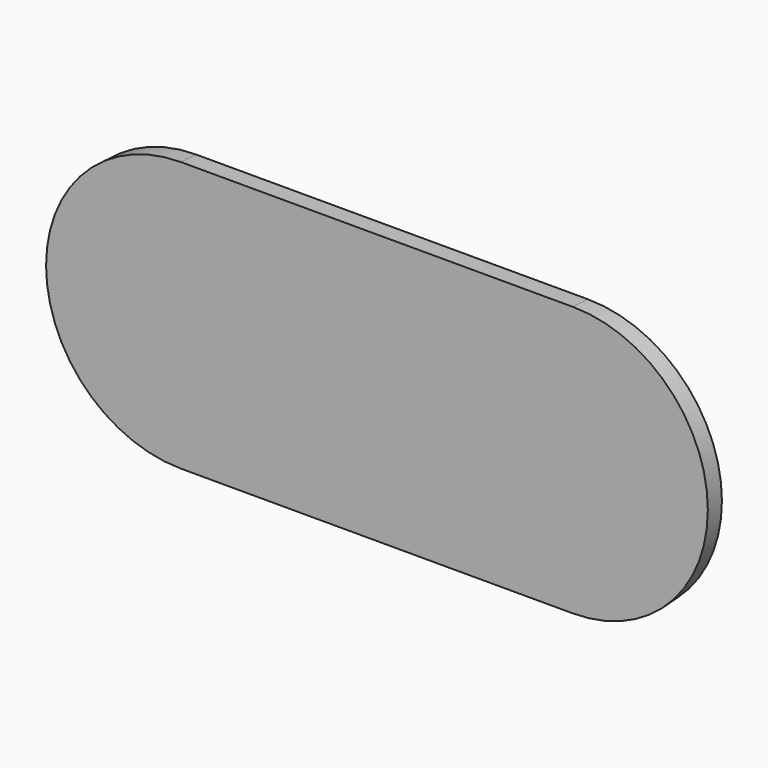
from build123d import *

# Parameters (mm, degrees)
F1_DEPTH = 4.7625
F1_TAPER = -3


# Not quite as in the source:
# - a length typed as a fraction of an inch, garbled in the dataset ("3 / 203.2 mm" for 3/8 in), is restored


with BuildPart() as f1:
    # F0 (on Front) → F1 (new body)
    with BuildSketch(Plane.XZ):
        with BuildLine():
            Line((0, 33.8334292173), (-49.4827702641, 33.8334292173))
            ThreePointArc((-49.4827702641, 33.8334292173), (-83.3161994815, 0), (-49.4827702641, -33.8334292173))
            Line((-49.4827702641, -33.8334292173), (0, -33.8334292173))
            Line((0, -33.8334292173), (49.4827702641, -33.8334292173))
            ThreePointArc((49.4827702641, -33.8334292173), (83.3161994815, 0), (49.4827702641, 33.8334292173))
            Line((49.4827702641, 33.8334292173), (0, 33.8334292173))
        make_face()
    extrude(amount=F1_DEPTH, taper=F1_TAPER)


solid = f1.part
